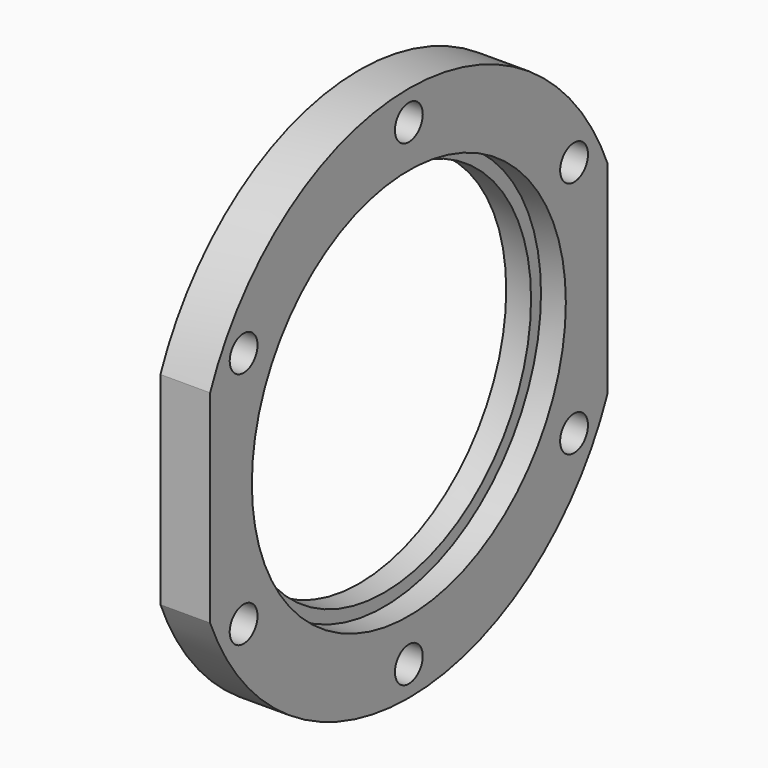
from build123d import *

# Parameters (mm, degrees)
F0_W            = 10
F0_H            = 17
F2_R            = 3.5
F3_DEPTH        = 10.001
F3_COPIES_COUNT = 6
F5_DEPTH        = 10.001
F6_R            = 39.5
F6_R_2          = 37
F7_DEPTH        = 5


# Not quite as in the source:
# - a pattern or mirror of a feature is missing from the dataset's text; its kind, count and spacing are read off the source's solid


with BuildPart() as f1:
    # F0 (on Front) → F1 (revolve)
    with BuildSketch(Plane.XZ):
        with Locations((5, 45.5)):
            Rectangle(F0_W, F0_H)
    revolve(axis=Axis((-28.7704151153, 0, 0), (-1, 0, 0)))

    # F2 (on face) → F3 (cut, through all)
    with BuildSketch(Plane(origin=(0, 0, 0), x_dir=(0, -1, 0), z_dir=(-1, 0, 0))):
        with Locations((41.5692193817, 24)):
            Circle(F2_R)
    f3 = extrude(amount=-F3_DEPTH, mode=Mode.SUBTRACT)

    # F3_copies: F3 ×6 about axis
    f3_copies_axis = Axis((0, 0, 0), (1, 0, 0))
    for i in range(1, F3_COPIES_COUNT):
        add(f3.rotate(f3_copies_axis, i * 360 / F3_COPIES_COUNT), mode=Mode.SUBTRACT)

    # F4 (on face) → F5 (cut, through all)
    with BuildSketch(Plane(origin=(0, 0, 0), x_dir=(0, -1, 0), z_dir=(-1, 0, 0))):
        with BuildLine():
            Line((-50, -20.3960780544), (-50, 20.3960780544))
            ThreePointArc((-50, 20.3960780544), (-54, 0), (-50, -20.3960780544))
        make_face()
        with BuildLine():
            ThreePointArc((54, 0), (52.990565198, 10.3923048454), (50, 20.3960780544))
            Line((50, 20.3960780544), (50, -20.3960780544))
            ThreePointArc((50, -20.3960780544), (52.990565198, -10.3923048454), (54, 0))
        make_face()
    extrude(amount=-F5_DEPTH, mode=Mode.SUBTRACT)

    # F6 (on face) → F7 (cut)
    with BuildSketch(Plane.YZ.offset(10)):
        Circle(F6_R)
        Circle(F6_R_2, mode=Mode.SUBTRACT)
    extrude(amount=-F7_DEPTH, mode=Mode.SUBTRACT)


solid = f1.part
